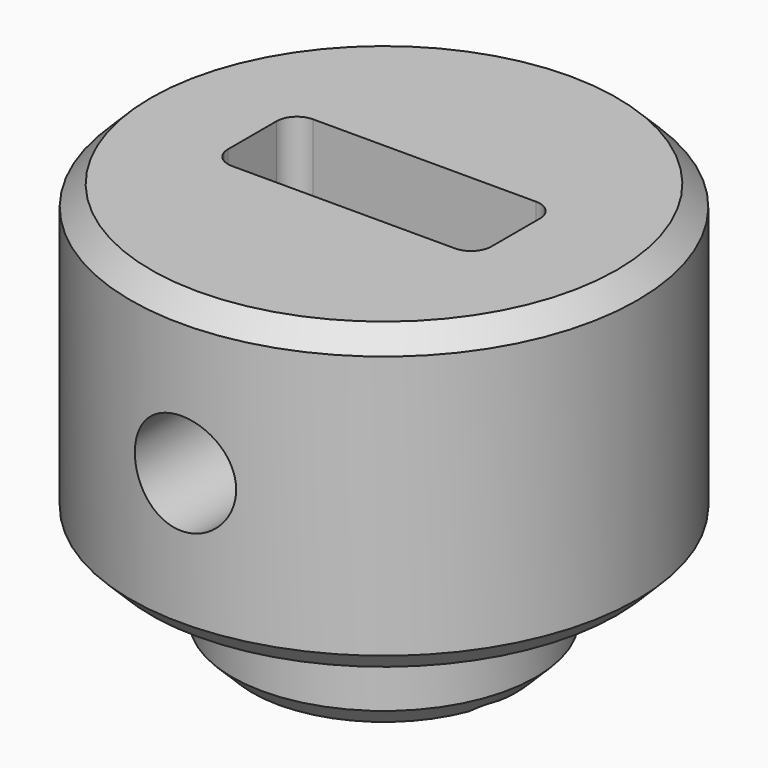
from build123d import *

# Parameters (mm, degrees)
F0_R     = 2.5
F1_DEPTH = 3
F2_R     = 1.5
F3_DEPTH = 1
F5_R     = 0.5
F6_DEPTH = 7.501
F7_W     = 2.6
F7_H     = 1
F8_DEPTH = 4.001
F9_R     = 0.2


# Not quite as in the source:
# - a fillet or chamfer that OpenCascade refuses, or shapes differently, is made with other operations: its cross-section is extruded or revolved along the edge and cut away or added


with BuildPart() as f1:
    # F0 (on Top) → F1 (new body)
    with BuildSketch(Plane.XY):
        Circle(F0_R)
    extrude(amount=F1_DEPTH)

    # F2 (on face) → F3 (join)
    with BuildSketch(Plane(origin=(0, 0, 0), x_dir=(1, 0, 0), z_dir=(0, 0, -1))):
        Circle(F2_R)
    extrude(amount=F3_DEPTH)

    # F5 (on offset) → F6 (cut, through all)
    with BuildSketch(Plane.XZ.offset(5)):
        with Locations((0, 1.5)):
            Circle(F5_R)
    extrude(amount=-F6_DEPTH, mode=Mode.SUBTRACT)

    # F7 (on face) → F8 (cut, through all)
    with BuildSketch(Plane.XY.offset(3)):
        Rectangle(F7_W, F7_H)
    extrude(amount=-F8_DEPTH, mode=Mode.SUBTRACT)

    # F9
    f9_edges = [f1.edges().sort_by_distance(p)[0] for p in [
        (-1.3, 0.5, 1),
        (-1.3, -0.5, 1),
        (1.3, -0.5, 1),
        (1.3, 0.5, 1),
    ]]
    fillet(f9_edges, radius=F9_R)

    # F10: chamfer of 0.2 on 3 edges, made by hand

    # F10_s1 → F10_t2 (revolve, cut)
    with BuildSketch(Plane.XZ):
        Polygon((2.3, 3), (2.5, 2.8), (2.5, 3), align=None)
    revolve(axis=Axis((0, 0, 3), (0, 0, 1)), mode=Mode.SUBTRACT)

    # F10_s3 → F10_t4 (revolve, cut)
    with BuildSketch(Plane.XZ):
        Polygon((2.5, 0.2), (2.3, 0), (2.5, 0), align=None)
    revolve(axis=Axis((0, 0, 0), (0, 0, 1)), mode=Mode.SUBTRACT)

    # F10_s5 → F10_t6 (revolve, cut)
    with BuildSketch(Plane.XZ):
        Polygon((1.3, -1), (1.5, -0.8), (1.5, -1), align=None)
    revolve(axis=Axis((0, 0, -1), (0, 0, -1)), mode=Mode.SUBTRACT)


solid = f1.part
